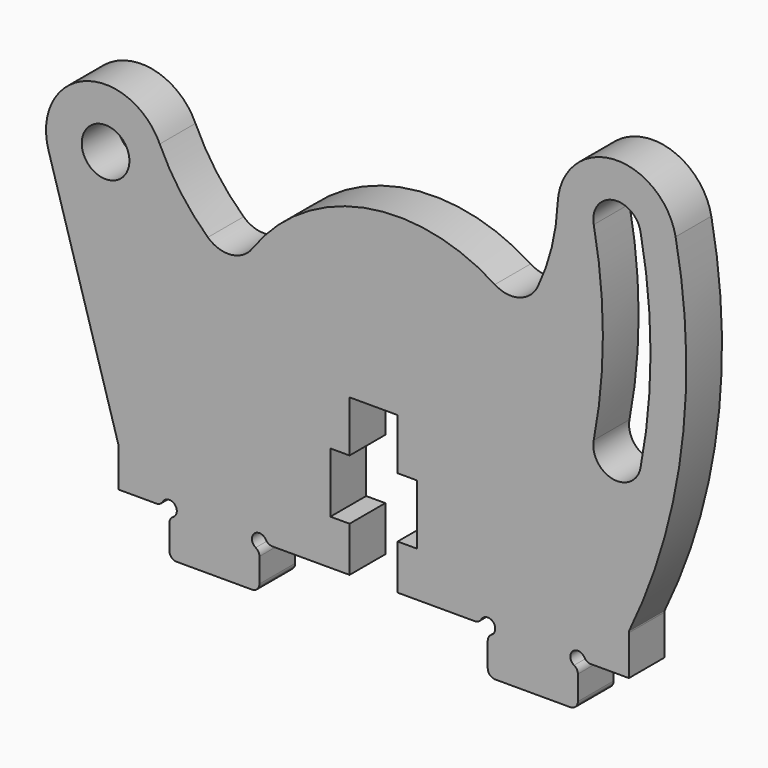
from build123d import *

# Parameters (mm, degrees)
F0_R     = 1.6
F1_DEPTH = 3


# Not quite as in the source:
# - ends of sketch curves that miss each other by under 0.0002 mm in the source are joined


with BuildPart() as f1:
    # F0 (on Front) → F1 (new body)
    with BuildSketch(Plane.XZ):
        with BuildLine():
            ThreePointArc((-10.6282638986, 3.1898001668), (-12.4668430477, 5.2626032061), (-13.8612036619, 7.6568972993))
            ThreePointArc((-13.8612036619, 7.6568972993), (-18.9011019651, 9.7424118848), (-21.335831, 4.861629))
            Line((-21.335831, 4.861629), (-16.648169, -10.991964))
            Line((-16.648169, -10.991964), (-16.648169, -13.674139))
            Line((-16.648169, -13.674139), (-14.092108, -13.6741314818))
            ThreePointArc((-14.092108, -13.6741314818), (-13.8399289655, -13.6065603025), (-13.6553211195, -13.4219524128))
            ThreePointArc((-13.6553211195, -13.4219524128), (-12.8619020996, -13.3175012704), (-12.9663588806, -14.1109235459))
            ThreePointArc((-12.9663588806, -14.1109235459), (-13.1509652395, -14.295530508), (-13.2185364188, -14.5477095425))
            Line((-13.2185364188, -14.5477095425), (-13.2185364188, -16.174139))
            ThreePointArc((-13.2185364188, -16.174139), (-13.0720898094, -16.5276923906), (-12.7185364188, -16.674139))
            Line((-12.7185364188, -16.674139), (-7.66624, -16.674139))
            ThreePointArc((-7.66624, -16.674139), (-7.3126880282, -16.5276923906), (-7.1662414188, -16.174139))
            Line((-7.1662414188, -16.174139), (-7.1662414188, -14.547714))
            ThreePointArc((-7.1662414188, -14.547714), (-7.2338128147, -14.2955345905), (-7.4184212378, -14.1109266865))
            ThreePointArc((-7.4184212378, -14.1109266865), (-7.522878567, -13.3175058971), (-6.7294565149, -13.4219591693))
            ThreePointArc((-6.7294565149, -13.4219591693), (-6.5448489948, -13.6065653787), (-6.2926709268, -13.674136))
            Line((-6.2926709268, -13.674136), (-1.113951, -13.674139))
            Line((-1.113951, -13.674139), (-1.113951, -10.64802))
            Line((-1.113951, -10.64802), (-2.400059, -10.64802))
            Line((-2.400059, -10.64802), (-2.400059, -6.613128))
            Line((-2.400059, -6.613128), (-1.113951, -6.613128))
            Line((-1.113951, -6.613128), (-1.113951, -3.174139))
            Line((-1.113951, -3.174139), (2.113951, -3.174141))
            Line((2.113951, -3.174141), (2.113951, -6.613128))
            Line((2.113951, -6.613128), (3.400058, -6.613128))
            Line((3.400058, -6.613128), (3.400059, -10.64802))
            Line((3.400059, -10.64802), (2.113951, -10.64802))
            Line((2.113951, -10.64802), (2.113951, -13.674139))
            Line((2.113951, -13.674139), (7.292668, -13.6741438699))
            ThreePointArc((7.292668, -13.6741438699), (7.5448470345, -13.6065678207), (7.7294548805, -13.421959931))
            ThreePointArc((7.7294548805, -13.421959931), (8.5228769619, -13.3175030381), (8.418420181, -14.1109253135))
            ThreePointArc((8.418420181, -14.1109253135), (8.2338115208, -14.295533374), (8.16624, -14.547713))
            Line((8.16624, -14.547713), (8.1662414188, -16.174139))
            ThreePointArc((8.1662414188, -16.174139), (8.3126866094, -16.5276923906), (8.66624, -16.674139))
            Line((8.66624, -16.674139), (13.718535, -16.674139))
            ThreePointArc((13.718535, -16.674139), (14.0720883906, -16.5276923906), (14.218535, -16.174139))
            Line((14.218535, -16.174139), (14.2185364188, -14.547713))
            ThreePointArc((14.2185364188, -14.547713), (14.1509638207, -14.2955339655), (13.966355931, -14.1109261195))
            ThreePointArc((13.966355931, -14.1109261195), (13.8618988613, -13.3175032148), (14.6553213135, -13.421959819))
            ThreePointArc((14.6553213135, -13.421959819), (14.8399289655, -13.6065678207), (15.092108, -13.674139))
            Line((15.092108, -13.674139), (17.648169, -13.6741498688))
            Line((17.648169, -13.6741498688), (17.648169, -10.991964))
            ThreePointArc((17.648169, -10.991964), (17.6480727307, -10.9478940797), (17.6477839247, -10.9038250007))
            Line((17.6477839247, -10.9038250007), (17.648169, -10.904063))
            ThreePointArc((17.648169, -10.904063), (21.1804529898, 1.0136018582), (20.7834599948, 13.437375999))
            ThreePointArc((20.7834599948, 13.437375999), (16.5617773272, 16.6632341642), (12.8608694009, 12.8511420265))
            ThreePointArc((12.8608694009, 12.8511420265), (12.4649591094, 10.1088544895), (11.5367438755, 7.4982410587))
            ThreePointArc((11.5367438755, 7.4982410587), (10.2794941976, 6.4290215203), (8.6465971955, 6.6689263042))
            ThreePointArc((8.6465971955, 6.6689263042), (-0.1307148674, 8.353355038), (-7.6378988754, 3.5035408071))
            ThreePointArc((-7.6378988754, 3.5035408071), (-9.062025187, 2.6694105221), (-10.6282638986, 3.1898001668))
        make_face()
        with Locations((-17.5000000032, 5.995824999)):
            Circle(F0_R, mode=Mode.SUBTRACT)
        with BuildLine():
            ThreePointArc((18.4275548403, 12.979433969), (19.0999998798, 5.9958249766), (18.4275548403, -0.9877840157))
            ThreePointArc((18.4275548491, -0.9877839707), (16.5516572505, -2.2530936185), (15.2863477145, -0.3771959445))
            ThreePointArc((15.2863477057, -0.3771959895), (15.8999998798, 5.9958244858), (15.286347893, 12.3688449792))
            ThreePointArc((15.286347905, 12.3688449179), (16.5516567719, 14.2447434618), (18.4275548522, 12.9794339076))
        make_face(mode=Mode.SUBTRACT)
    extrude(amount=F1_DEPTH)


solid = f1.part
